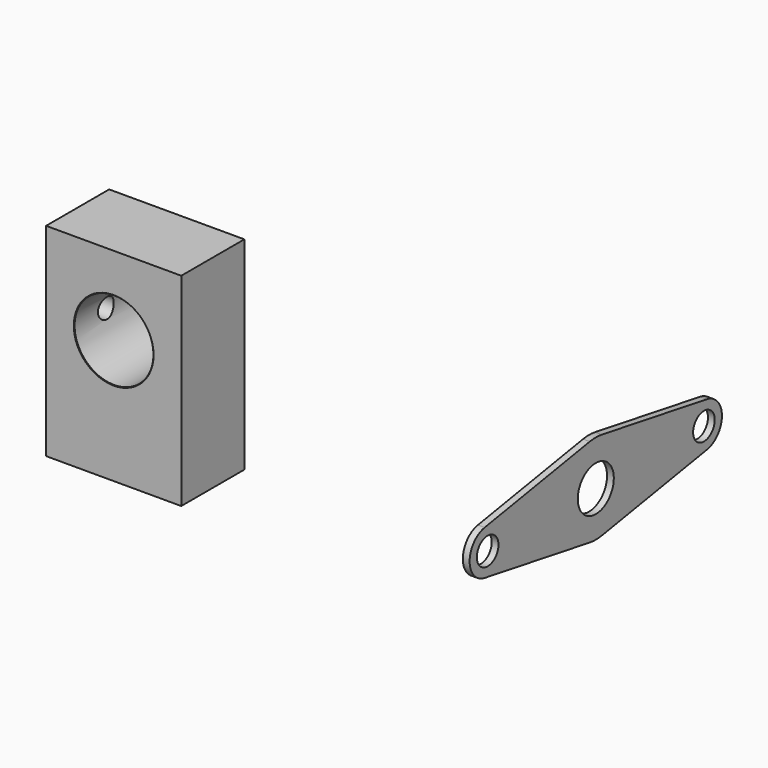
from build123d import *

# Parameters (mm, degrees)
F0_W           = 60
F0_H           = 90
F0_R           = 17.5
F1_DEPTH       = 17.5
F3_D           = 8.8
F3_DEPTH       = 15
F3_CBORE_D     = 17.25
F3_CBORE_DEPTH = 5
F3_TIP         = 2.6437867237
F4_SIZE        = 0.2
F5_R           = 6
F5_R_2         = 10
F6_DEPTH       = 3


with BuildPart() as f1:
    # F0 (on Front) → F1 (new body, symmetric)
    with BuildSketch(Plane.XZ):
        with Locations((-200, -10)):
            Rectangle(F0_W, F0_H)
        with Locations((-200, 0)):
            Circle(F0_R, mode=Mode.SUBTRACT)
    extrude(amount=F1_DEPTH, both=True)

    # F3
    with Locations(Plane(origin=(-230, 0, 0), x_dir=(0, -1, 0), z_dir=(-1, 0, 0))):
        with Locations((0, 0)):
            CounterBoreHole(F3_D / 2, F3_CBORE_D / 2, F3_CBORE_DEPTH, depth=F3_DEPTH)
            with Locations((0, 0, -(F3_DEPTH + F3_TIP / 2))):  # 118° drill point
                Cone(0, F3_D / 2, F3_TIP, mode=Mode.SUBTRACT)

    # F4
    f4_edges = [f1.edges().sort_by_distance(p)[0] for p in [
        (-217.5, -17.5, 0),
        (-217.5, 17.5, 0),
        (-230, 8.625, 0),
    ]]
    chamfer(f4_edges, length=F4_SIZE)


with BuildPart() as f6:
    # F5 (on Right) → F6 (new body)
    with BuildSketch(Plane.YZ):
        with BuildLine():
            Line((61.6666666667, 9.8601329718), (3.3333333333, 19.7202659437))
            ThreePointArc((3.3333333333, 19.7202659437), (0, 20), (-3.3333333333, 19.7202659437))
            Line((-3.3333333333, 19.7202659437), (-61.6666666667, 9.8601329718))
            ThreePointArc((-61.6666666667, 9.8601329718), (-70, 0), (-61.6666666667, -9.8601329718))
            Line((-61.6666666667, -9.8601329718), (-3.3333333333, -19.7202659437))
            ThreePointArc((-3.3333333333, -19.7202659437), (0, -20), (3.3333333333, -19.7202659437))
            Line((3.3333333333, -19.7202659437), (61.6666666667, -9.8601329718))
            ThreePointArc((61.6666666667, -9.8601329718), (70, 0), (61.6666666667, 9.8601329718))
        make_face()
        with Locations((-60, 0)):
            Circle(F5_R, mode=Mode.SUBTRACT)
        Circle(F5_R_2, mode=Mode.SUBTRACT)
        with Locations((60, 0)):
            Circle(F5_R, mode=Mode.SUBTRACT)
    extrude(amount=-F6_DEPTH)


solid = Compound([f1.part, f6.part])
